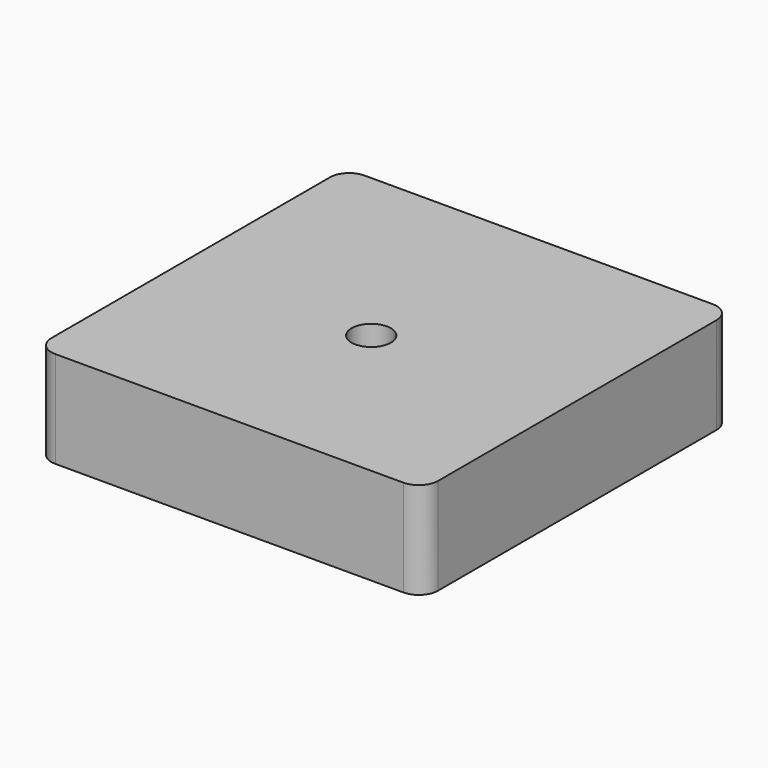
from build123d import *

# Parameters (mm, degrees)
F0_W     = 101.6
F0_H     = 101.6
F1_DEPTH = 25.4
F2_R     = 5.08
F3_R     = 5.08
F4_R     = 5.08
F5_R     = 5.08
F7_D     = 10.31875


# Not quite as in the source:
# - a length typed as a fraction of an inch, garbled in the dataset ("3 / 203.2 mm" for 3/8 in), is restored


with BuildPart() as f1:
    # F0 (on Top) → F1 (new body)
    with BuildSketch(Plane.XY):
        with Locations((-24.6530866301, 19.163233228)):
            Rectangle(F0_W, F0_H)
    extrude(amount=F1_DEPTH)

    # F2
    f2_edges = [f1.edges().sort_by_distance(p)[0] for p in [
        (-75.453087, 69.963233, 12.7),
    ]]
    fillet(f2_edges, radius=F2_R)

    # F3
    f3_edges = [f1.edges().sort_by_distance(p)[0] for p in [
        (-75.453087, -31.636767, 12.7),
    ]]
    fillet(f3_edges, radius=F3_R)

    # F4
    f4_edges = [f1.edges().sort_by_distance(p)[0] for p in [
        (26.146913, 69.963233, 12.7),
    ]]
    fillet(f4_edges, radius=F4_R)

    # F5
    f5_edges = [f1.edges().sort_by_distance(p)[0] for p in [
        (26.146913, -31.636767, 12.7),
    ]]
    fillet(f5_edges, radius=F5_R)

    # F7 (through all)
    with Locations(Plane.XY.offset(25.4)):
        with Locations((-24.9434951693, 15.3265725821)):
            Hole(F7_D / 2)


solid = f1.part
